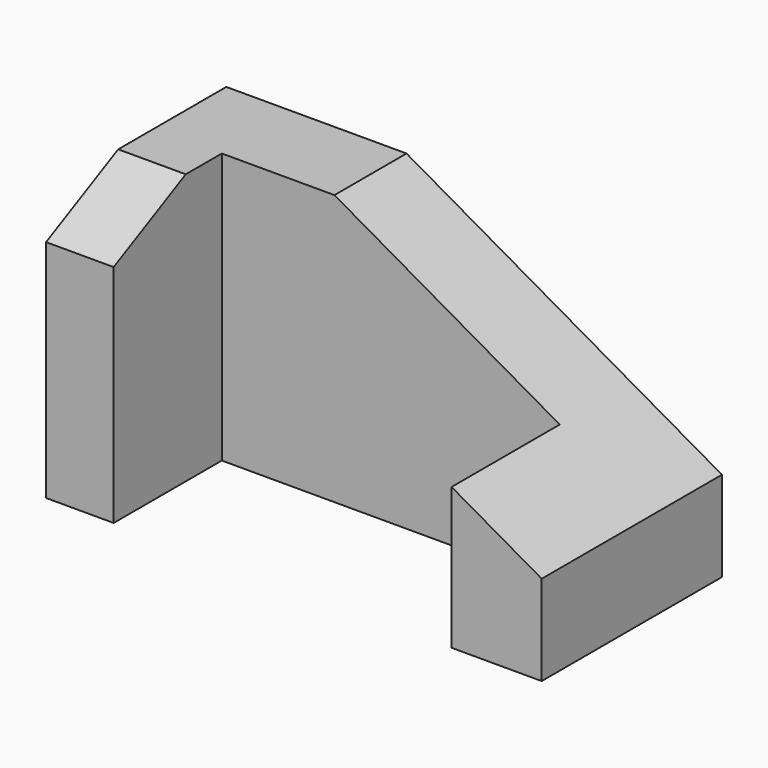
from build123d import *

# Parameters (mm, degrees)
F1_DEPTH = 60
F3_DEPTH = 15
F5_DEPTH = 60


# Not quite as in the source:
# - a feature names something its author has since deleted; it is built from what else it names


with BuildPart() as f1:
    # F0 (on Top) → F1 (new body)
    with BuildSketch(Plane.XY):
        Polygon((55, 25), (-55, 25), (-55, -25), (-40, -25), (-40, 5), (35, 5), (35, -25), (55, -25), align=None)
    extrude(amount=F1_DEPTH)

    # F2 (on face) → F3 (cut)
    with BuildSketch(Plane(origin=(-55, 0, 0), x_dir=(0, -1, 0), z_dir=(-1, 0, 0))):
        Polygon((25, 60), (5, 60), (25, 50), align=None)
    extrude(amount=-F3_DEPTH, mode=Mode.SUBTRACT)

    # F4 (on face) → F5 (cut)
    with BuildSketch(Plane(origin=(0, 25, 0), x_dir=(-1, 0, 0), z_dir=(0, 1, 0))):
        Polygon((15, 60), (-55, 60), (-55, 20), align=None)
    extrude(amount=-F5_DEPTH, mode=Mode.SUBTRACT)


solid = f1.part
